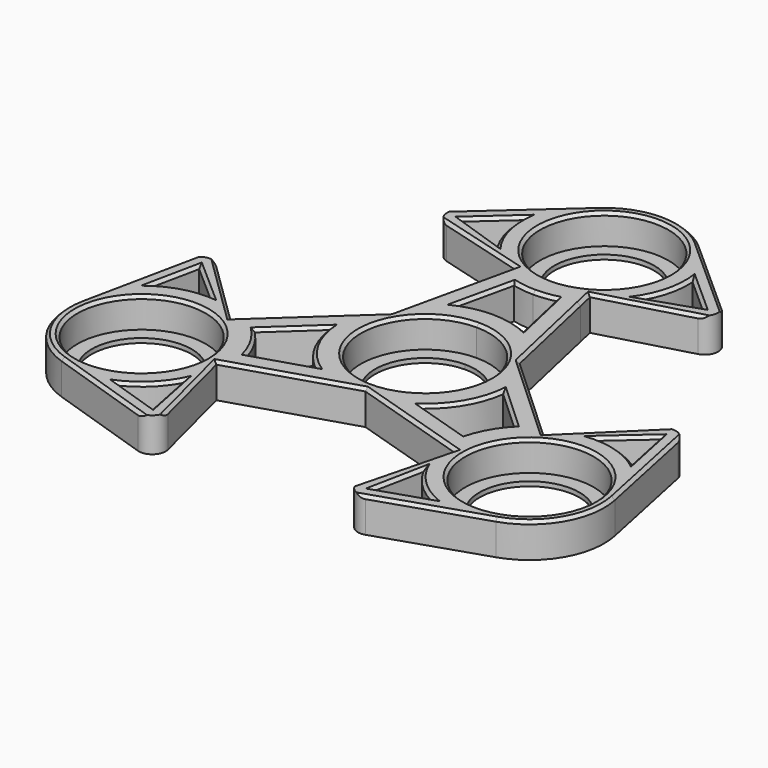
from build123d import *

# Parameters (mm, degrees)
F1_DEPTH    = 0.762
F0_R        = 10.922
F0_R_2      = 8.509
F2_DEPTH    = 5.842
F3_SIZE     = 0.508
F4_T1_DEPTH = 26.2029203158


# Not quite as in the source:
# - a fillet or chamfer that OpenCascade refuses, or shapes differently, is made with other operations: its cross-section is extruded or revolved along the edge and cut away or added
# - a feature names something its author has since deleted; it is built from what else it names


with BuildPart() as f1:
    # F0 (on Top) → F1 (new body)
    with BuildSketch(Plane.XY):
        with BuildLine():
            ThreePointArc((0, 10.922), (-7.7230202641, -7.7230202641), (10.922, 0))
            ThreePointArc((10.922, 0), (7.7230202641, 7.7230202641), (0, 10.922))
        make_face()
        with BuildLine():
            ThreePointArc((8.509, 0), (-6.0167716011, -6.0167716011), (0, 8.509))
            ThreePointArc((0, 8.509), (6.0167716011, 6.0167716011), (8.509, 0))
        make_face(mode=Mode.SUBTRACT)
    extrude(amount=F1_DEPTH)



with BuildPart() as f1b:
    # F0 (on Top) → F1, piece 2 (new body)
    with BuildSketch(Plane.XY):
        with Locations((32.9955678842, -19.05)):
            Circle(F0_R)
        with Locations((32.9955678842, -19.05)):
            Circle(F0_R_2, mode=Mode.SUBTRACT)
    extrude(amount=F1_DEPTH)


with BuildPart() as f1c:
    # F0 (on Top) → F1, piece 3 (new body)
    with BuildSketch(Plane.XY):
        with BuildLine():
            ThreePointArc((10.922, 38.1), (-7.7230202641, 45.8230202641), (0, 27.178))
            ThreePointArc((0, 27.178), (7.7230202641, 30.3769797359), (10.922, 38.1))
        make_face()
        with BuildLine():
            ThreePointArc((8.509, 38.1), (6.0167716011, 32.0832283989), (0, 29.591))
            ThreePointArc((0, 29.591), (-6.0167716011, 44.1167716011), (8.509, 38.1))
        make_face(mode=Mode.SUBTRACT)
    extrude(amount=F1_DEPTH)


with BuildPart() as f1d:
    # F0 (on Top) → F1, piece 4 (new body)
    with BuildSketch(Plane.XY):
        with Locations((-32.9955678842, -19.05)):
            Circle(F0_R)
        with Locations((-32.9955678842, -19.05)):
            Circle(F0_R_2, mode=Mode.SUBTRACT)
    extrude(amount=F1_DEPTH)


with BuildPart() as f1_1:
    add(f1.part)

    add(f1b.part)  # F2 merges F1b

    add(f1c.part)  # F2 merges F1c

    add(f1d.part)  # F2 merges F1d
    # F0 (on Top) → F2 (join)
    with BuildSketch(Plane.XY):
        with BuildLine():
            Line((25.4, 32.4302427471), (8.4636048701, 47.5687587678))
            ThreePointArc((8.4636048701, 47.5687587678), (0, 50.8), (-8.4636048701, 47.5687587678))
            Line((-8.4636048701, 47.5687587678), (-25.4, 32.4302427471))
            Line((-25.4, 32.4302427471), (-6.35, 27.1014773719))
            Line((-6.35, 27.1014773719), (-6.9723232388, 24.3233631966))
            Line((-6.9723232388, 24.3233631966), (-10.9985226281, 6.35))
            Line((-10.9985226281, 6.35), (-26.6455678842, -8.0514773719))
            Line((-26.6455678842, -8.0514773719), (-40.7854140699, 5.7819238826))
            Line((-40.7854140699, 5.7819238826), (-45.4275559545, -16.4546825588))
            ThreePointArc((-45.4275559545, -16.4546825588), (-43.9940905122, -25.4), (-36.9639510844, -31.114076209))
            Line((-36.9639510844, -31.114076209), (-15.3854140699, -38.2121666297))
            Line((-15.3854140699, -38.2121666297), (-20.2955678842, -19.05))
            Line((-20.2955678842, -19.05), (0, -12.7))
            Line((0, -12.7), (20.2955678842, -19.05))
            Line((20.2955678842, -19.05), (15.3854140699, -38.2121666297))
            Line((15.3854140699, -38.2121666297), (36.9639510844, -31.114076209))
            ThreePointArc((36.9639510844, -31.114076209), (43.9940905122, -25.4), (45.4275559545, -16.4546825588))
            Line((45.4275559545, -16.4546825588), (40.7854140699, 5.7819238826))
            Line((40.7854140699, 5.7819238826), (26.6455678842, -8.0514773719))
            Line((26.6455678842, -8.0514773719), (10.9985226281, 6.35))
            Line((10.9985226281, 6.35), (6.9723232388, 24.3233631966))
            Line((6.9723232388, 24.3233631966), (6.35, 27.1014773719))
            Line((6.35, 27.1014773719), (25.4, 32.4302427471))
        make_face()
        with Locations((-32.9955678842, -19.05)):
            Circle(F0_R, mode=Mode.SUBTRACT)
        with BuildLine():
            Line((-18.7647342027, -34.4713298417), (-26.6406054915, -31.8806237845))
            ThreePointArc((-26.6406054915, -31.8806237845), (-23.1036446868, -29.4018263687), (-20.4667802357, -25.9810846026))
            Line((-20.4667802357, -25.9810846026), (-18.7647342027, -34.4713298417))
        make_face(mode=Mode.SUBTRACT)
        with BuildLine():
            Line((-40.932005297, -7.1326422852), (-39.2370618115, 0.9864096878))
            Line((-39.2370618115, 0.9864096878), (-32.733650082, -4.7342096699))
            ThreePointArc((-32.733650082, -4.7342096699), (-37.0158517754, -5.3078105404), (-40.932005297, -7.1326422852))
        make_face(mode=Mode.SUBTRACT)
        with BuildLine():
            Line((-22.0797985411, -8.6046126406), (-14.7828681473, -1.888547324))
            ThreePointArc((-14.7828681473, -1.888547324), (-12.9063880014, -7.4515065869), (-9.0269640325, -11.8580656943))
            Line((-9.0269640325, -11.8580656943), (-18.491712407, -14.8193601267))
            ThreePointArc((-18.491712407, -14.8193601267), (-19.9114132275, -11.4958597868), (-22.0797985411, -8.6046126406))
        make_face(mode=Mode.SUBTRACT)
        with BuildLine():
            Line((26.6430520636, -31.8818352724), (18.7642750576, -34.4734971425))
            Line((18.7642750576, -34.4734971425), (20.466770882, -25.9810676946))
            ThreePointArc((20.466770882, -25.9810676946), (23.1046246541, -29.40276271), (26.6430520636, -31.8818352724))
        make_face(mode=Mode.SUBTRACT)
        with Locations((32.9955678842, -19.05)):
            Circle(F0_R, mode=Mode.SUBTRACT)
        with BuildLine():
            Line((18.491712407, -14.8193601267), (9.0269640325, -11.8580656943))
            ThreePointArc((9.0269640325, -11.8580656943), (12.9063880014, -7.4515065869), (14.7828681473, -1.888547324))
            Line((14.7828681473, -1.888547324), (22.0797985411, -8.6046126406))
            ThreePointArc((22.0797985411, -8.6046126406), (19.9114132275, -11.4958597868), (18.491712407, -14.8193601267))
        make_face(mode=Mode.SUBTRACT)
        with BuildLine():
            ThreePointArc((0, 10.922), (7.7230202641, 7.7230202641), (10.922, 0))
            ThreePointArc((10.922, 0), (-7.7230202641, -7.7230202641), (0, 10.922))
        make_face(mode=Mode.SUBTRACT)
        with BuildLine():
            Line((39.2354144465, 0.984928406), (40.9297328316, -7.1311292356))
            ThreePointArc((40.9297328316, -7.1311292356), (37.0145508963, -5.3074300344), (32.7336694016, -4.7342093164))
            Line((32.7336694016, -4.7342093164), (39.2354144465, 0.984928406))
        make_face(mode=Mode.SUBTRACT)
        with BuildLine():
            ThreePointArc((5.7559041148, 13.7466130184), (2.935459653, 14.6110532913), (0, 14.9030131737))
            ThreePointArc((0, 14.9030131737), (-2.935459653, 14.6110532913), (-5.7559041148, 13.7466130184))
            Line((-5.7559041148, 13.7466130184), (-3.5880861341, 23.4239727673))
            ThreePointArc((-3.5880861341, 23.4239727673), (-1.8070144527, 23.1001721274), (0, 22.9917195737))
            ThreePointArc((0, 22.9917195737), (1.8070144527, 23.1001721274), (3.5880861341, 23.4239727673))
            Line((3.5880861341, 23.4239727673), (5.7559041148, 13.7466130184))
        make_face(mode=Mode.SUBTRACT)
        with BuildLine():
            Line((-20.4706802438, 33.4864014357), (-14.2891273401, 39.0117530201))
            ThreePointArc((-14.2891273401, 39.0117530201), (-13.9109062095, 34.7092564031), (-12.2668891659, 30.7152939191))
            Line((-12.2668891659, 30.7152939191), (-20.4706802438, 33.4864014357))
        make_face(mode=Mode.SUBTRACT)
        with BuildLine():
            ThreePointArc((10.922, 38.1), (7.7230202641, 30.3769797359), (0, 27.178))
            ThreePointArc((0, 27.178), (-7.7230202641, 45.8230202641), (10.922, 38.1))
        make_face(mode=Mode.SUBTRACT)
        with BuildLine():
            Line((20.4727867539, 33.4870874547), (12.2668792, 30.7152773645))
            ThreePointArc((12.2668792, 30.7152773645), (13.9112271213, 34.7105732504), (14.2889532334, 39.0144775576))
            Line((14.2889532334, 39.0144775576), (20.4727867539, 33.4870874547))
        make_face(mode=Mode.SUBTRACT)
    extrude(amount=F2_DEPTH)

    # F3
    f3_edges = [f1_1.edges().sort_by_distance(p)[0] for p in [
        (43.106485, -5.336379, 5.842),
        (33.715491, -1.134777, 5.842),
        (18.822045, -0.850739, 5.842),
        (8.674261, 16.725739, 5.842),
        (15.875, 29.76586, 5.842),
        (16.931802, 39.999501, 5.842),
        (0, 50.8, 5.842),
        (-16.931802, 39.999501, 5.842),
        (-15.875, 29.76586, 5.842),
        (-8.674261, 16.725739, 5.842),
        (-18.822045, -0.850739, 5.842),
        (-33.715491, -1.134777, 5.842),
        (-43.106485, -5.336379, 5.842),
        (-43.994091, -25.4, 5.842),
        (-26.174683, -34.663121, 5.842),
        (-17.840491, -28.631083, 5.842),
        (-10.147784, -15.875, 5.842),
        (10.147784, -15.875, 5.842),
        (17.840491, -28.631083, 5.842),
        (26.174683, -34.663121, 5.842),
        (43.994091, -25.4, 5.842),
        (-43.917568, -19.05, 5.842),
        (-22.70267, -33.175977, 5.842),
        (-23.103645, -29.401826, 5.842),
        (-19.615757, -30.226207, 5.842),
        (-40.084534, -3.073116, 5.842),
        (-35.985356, -1.8739, 5.842),
        (-37.015852, -5.307811, 5.842),
        (-12.906388, -7.451507, 5.842),
        (-13.759338, -13.338713, 5.842),
        (-19.911413, -11.49586, 5.842),
        (-18.431333, -5.24658, 5.842),
        (23.104625, -29.402763, 5.842),
        (22.703664, -33.177666, 5.842),
        (19.615523, -30.227282, 5.842),
        (22.073568, -19.05, 5.842),
        (13.759338, -13.338713, 5.842),
        (12.906388, -7.451507, 5.842),
        (18.431333, -5.24658, 5.842),
        (19.911413, -11.49586, 5.842),
        (-10.922, 0, 5.842),
        (35.984542, -1.87464, 5.842),
        (40.082574, -3.0731, 5.842),
        (37.014551, -5.30743, 5.842),
        (4.671995, 18.585293, 5.842),
        (0, 14.903013, 5.842),
        (-4.671995, 18.585293, 5.842),
        (0, 22.99172, 5.842),
        (-17.379904, 36.249077, 5.842),
        (-13.910906, 34.709256, 5.842),
        (-16.368785, 32.100848, 5.842),
        (0, 49.022, 5.842),
        (17.38087, 36.250783, 5.842),
        (16.369833, 32.101182, 5.842),
        (13.911227, 34.710573, 5.842),
    ]]
    chamfer(f3_edges, length=F3_SIZE)

    # F4: fillet of radius 2.286 on 6 edges, made by hand

    # F4_s2 → F4_t1 (cut)
    with BuildSketch(Plane.XY.offset(-10.4344601579)):
        with BuildLine():
            ThreePointArc((-41.6383506506, 1.6962204431), (-40.0658224776, 3.4161310835), (-37.8019506719, 2.8631194083))
            Line((-37.8019506719, 2.8631194083), (-40.7854140699, 5.7819238826))
            Line((-40.7854140699, 5.7819238826), (-41.6383506506, 1.6962204431))
        make_face()
        with BuildLine():
            ThreePointArc((-22.2881453195, 35.2117592135), (-22.9913675398, 32.9899545474), (-21.3805094776, 31.3058898903))
            Line((-21.3805094776, 31.3058898903), (-25.4, 32.4302427471))
            Line((-25.4, 32.4302427471), (-22.2881453195, 35.2117592135))
        make_face()
        with BuildLine():
            ThreePointArc((21.3805094776, 31.3058898903), (22.9913675398, 32.9899545474), (22.2881453195, 35.2117592135))
            Line((22.2881453195, 35.2117592135), (25.4, 32.4302427471))
            Line((25.4, 32.4302427471), (21.3805094776, 31.3058898903))
        make_face()
        with BuildLine():
            ThreePointArc((41.6383506506, 1.6962204431), (40.0658224776, 3.4161310835), (37.8019506719, 2.8631194083))
            Line((37.8019506719, 2.8631194083), (40.7854140699, 5.7819238826))
            Line((40.7854140699, 5.7819238826), (41.6383506506, 1.6962204431))
        make_face()
        with BuildLine():
            ThreePointArc((19.3502053311, -36.9079796566), (17.0744549378, -36.4060856309), (16.4214411943, -34.1690092986))
            Line((16.4214411943, -34.1690092986), (15.3854140699, -38.2121666297))
            Line((15.3854140699, -38.2121666297), (19.3502053311, -36.9079796566))
        make_face()
        with BuildLine():
            ThreePointArc((-16.4214411943, -34.1690092986), (-17.0744549378, -36.4060856309), (-19.3502053311, -36.9079796566))
            Line((-19.3502053311, -36.9079796566), (-15.3854140699, -38.2121666297))
            Line((-15.3854140699, -38.2121666297), (-16.4214411943, -34.1690092986))
        make_face()
    extrude(amount=F4_T1_DEPTH, mode=Mode.SUBTRACT)


solid = f1_1.part
